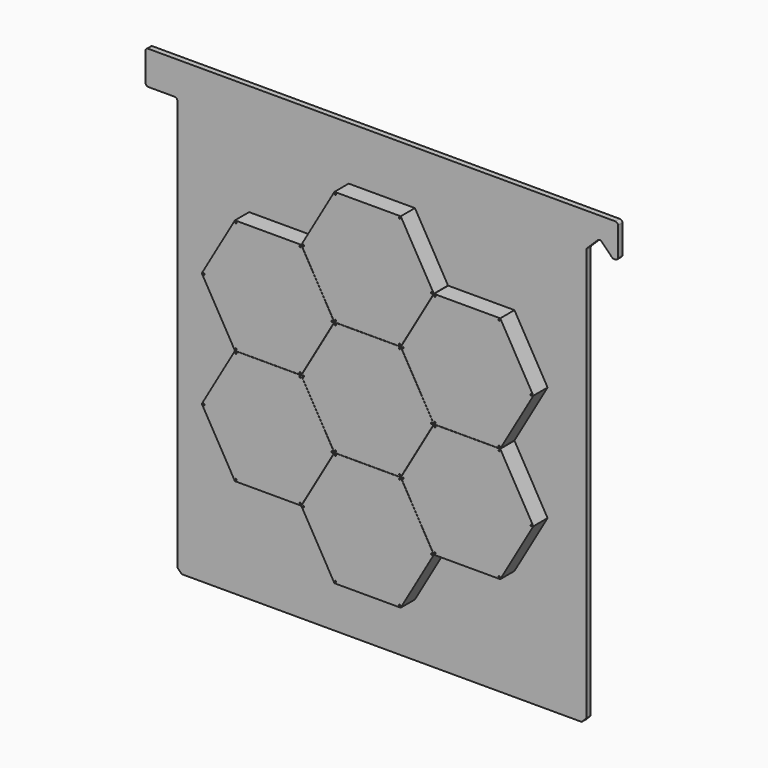
from build123d import *

# Parameters (mm, degrees)
F2_DEPTH = 6
F0_R     = 0.7500112
F0_R_2   = 0.7430174238
F3_DEPTH = 25.4


# Not quite as in the source:
# - ends of sketch curves that miss each other by under 0.0002 mm in the source are joined


with BuildPart() as f2:
    # F1 (on face) → F2 (new body)
    with BuildSketch(Plane.XZ):
        with BuildLine():
            Line((239.9250705835, 222.0849408719), (251.1754686974, 210.6445925623))
            ThreePointArc((251.1754686974, 210.6445925623), (252.1467535933, 209.9867437177), (253.2968294671, 209.755476289))
            Line((253.2968294671, 209.755476289), (254.8801768619, 209.755476289))
            ThreePointArc((254.8801768619, 209.755476289), (256.983999836, 210.6269082977), (257.8554318447, 212.7307312719))
            Line((257.8554318447, 212.7307312719), (257.8554318447, 243.475032761))
            ThreePointArc((257.8554318447, 243.475032761), (256.983999836, 245.5788557351), (254.8801768619, 246.4502877439))
            Line((254.8801768619, 246.4502877439), (-254.8801768619, 246.4502877439))
            ThreePointArc((-254.8801768619, 246.4502877439), (-256.983999836, 245.5788557351), (-257.8554318447, 243.475032761))
            Line((-257.8554318447, 243.475032761), (-257.8554318447, 212.7307312719))
            ThreePointArc((-257.8554318447, 212.7307312719), (-256.983999836, 210.6269082977), (-254.8801768619, 209.755476289))
            Line((-254.8801768619, 209.755476289), (-226.1193786946, 209.755476289))
            ThreePointArc((-226.1193786946, 209.755476289), (-224.0155557204, 208.8840442803), (-223.1441237117, 206.7802213062))
            Line((-223.1441237117, 206.7802213062), (-223.1441237117, -241.4915294391))
            Line((-223.1441237117, -241.4915294391), (-218.185365407, -246.4502877439))
            Line((-218.185365407, -246.4502877439), (218.185365407, -246.4502877439))
            Line((218.185365407, -246.4502877439), (223.1441237117, -241.4915294391))
            Line((223.1441237117, -241.4915294391), (223.1441237117, 208.5084705609))
            ThreePointArc((223.1441237117, 208.5084705609), (223.375391006, 209.658546114), (224.0332399627, 210.6298303616))
            Line((224.0332399627, 210.6298303616), (235.7175720959, 222.1201619404))
            ThreePointArc((235.7175720959, 222.1201619404), (237.8286155716, 222.9739529007), (239.9250705835, 222.0849408719))
        make_face()
        Polygon((72.2957914, 0), (36.1479084, -62.6100094), (-36.1479084, -62.6100094), (-72.2957914, 0), (-36.1479084, 62.6100094), (36.1479084, 62.6100094), align=None, mode=Mode.SUBTRACT)
    extrude(amount=F2_DEPTH)

    # F0 (on Front) → F3 (join)
    with BuildSketch(Plane.XZ):
        Polygon((36.1479084, -62.6100094), (72.2957914, 0), (36.1479084, 62.6100094), (-36.1479084, 62.6100094), (-72.2957914, 0), (-36.1479084, -62.6100094), align=None)
        with Locations((-34.993199, -60.609988)):
            Circle(F0_R, mode=Mode.SUBTRACT)
        with Locations((34.993199, -60.609988)):
            Circle(F0_R, mode=Mode.SUBTRACT)
        with Locations((-69.986398, 0)):
            Circle(F0_R, mode=Mode.SUBTRACT)
        with Locations((-34.993199, 60.609988)):
            Circle(F0_R, mode=Mode.SUBTRACT)
        with Locations((69.995796, 0)):
            Circle(F0_R_2, mode=Mode.SUBTRACT)
        with Locations((34.993199, 60.609988)):
            Circle(F0_R, mode=Mode.SUBTRACT)
        Polygon((72.47959348, -0.1061088931), (36.3364219227, -62.7188382077), (72.4890757311, -125.3261121412), (144.7848756936, -125.3206127679), (180.9280472508, -62.7078834532), (144.7753934424, -0.1006095197), align=None)
        with Locations((73.6436387774, -123.3260062512)):
            Circle(F0_R, mode=Mode.SUBTRACT)
        with Locations((143.6300274078, -123.3207069419)):
            Circle(F0_R, mode=Mode.SUBTRACT)
        with Locations((38.6458459563, -62.7186601398)):
            Circle(F0_R, mode=Mode.SUBTRACT)
        with Locations((73.6297421488, -2.0978761685)):
            Circle(F0_R_2, mode=Mode.SUBTRACT)
        with Locations((178.6186232172, -62.7080615211)):
            Circle(F0_R, mode=Mode.SUBTRACT)
        with Locations((143.6208303961, -2.1007154097)):
            Circle(F0_R, mode=Mode.SUBTRACT)
        Polygon((36.1478997424, -62.8259687739), (-36.1479168252, -62.8201722222), (-72.3008196697, -125.4272831471), (-36.1579567466, -188.0401906197), (36.1378598211, -188.0459871714), (72.2907626655, -125.4388762464), align=None)
        with Locations((-35.0030869921, -186.0402618087)):
            Circle(F0_R, mode=Mode.SUBTRACT)
        with Locations((-69.9914262771, -125.4274683102)):
            Circle(F0_R, mode=Mode.SUBTRACT)
        with Locations((-34.9933677872, -64.8202861983)):
            Circle(F0_R, mode=Mode.SUBTRACT)
        with Locations((34.983310783, -186.0458731952)):
            Circle(F0_R, mode=Mode.SUBTRACT)
        with Locations((69.9907672729, -125.4386918368)):
            Circle(F0_R_2, mode=Mode.SUBTRACT)
        with Locations((34.9930299879, -64.8258975849)):
            Circle(F0_R, mode=Mode.SUBTRACT)
        Polygon((-36.3200081195, -62.7093545109), (-72.4588066668, -0.0941010816), (-144.7546060688, -0.0835525132), (-180.91163233, -62.6883013644), (-144.7728337827, -125.3035547937), (-72.4770343807, -125.3141033621), align=None)
        with Locations((-143.6225460101, -123.3118678504)):
            Circle(F0_R_2, mode=Mode.SUBTRACT)
        with Locations((-73.6314577352, -123.3139168414)):
            Circle(F0_R, mode=Mode.SUBTRACT)
        with Locations((-178.6022083144, -62.6886407243)):
            Circle(F0_R, mode=Mode.SUBTRACT)
        with Locations((-143.6001827143, -2.0837390339)):
            Circle(F0_R, mode=Mode.SUBTRACT)
        with Locations((-38.6294321351, -62.709015151)):
            Circle(F0_R, mode=Mode.SUBTRACT)
        with Locations((-73.6137946247, -2.0939262472)):
            Circle(F0_R, mode=Mode.SUBTRACT)
        Polygon((-72.4855936704, 0.1095682125), (-36.3446929989, 62.7236083401), (-72.4996174478, 125.3295710344), (-144.7954171632, 125.3214496097), (-180.9363178347, 62.7074094821), (-144.7813933858, 0.1014467878), align=None)
        with Locations((-143.6269028809, 2.1015945506)):
            Circle(F0_R, mode=Mode.SUBTRACT)
        with Locations((-178.626893809, 62.707671309)):
            Circle(F0_R, mode=Mode.SUBTRACT)
        with Locations((-73.6405144887, 2.1094321527)):
            Circle(F0_R, mode=Mode.SUBTRACT)
        with Locations((-38.6541170246, 62.7233465131)):
            Circle(F0_R, mode=Mode.SUBTRACT)
        with Locations((-143.645196257, 123.3297240496)):
            Circle(F0_R_2, mode=Mode.SUBTRACT)
        with Locations((-73.6541079527, 123.3294232716)):
            Circle(F0_R, mode=Mode.SUBTRACT)
        Polygon((-36.1479091406, 62.8225415071), (36.1479076577, 62.8230453272), (72.2953543359, 125.4333066355), (36.1470350159, 188.0430641241), (-36.1487817824, 188.0425603041), (-72.2962284606, 125.4322989958), align=None)
        with Locations((-34.9932136785, 64.8225709541)):
            Circle(F0_R, mode=Mode.SUBTRACT)
        with Locations((-69.9868350606, 125.4323150896)):
            Circle(F0_R, mode=Mode.SUBTRACT)
        with Locations((-34.9940584445, 186.0425469512)):
            Circle(F0_R, mode=Mode.SUBTRACT)
        with Locations((34.9931843198, 64.8230586801)):
            Circle(F0_R, mode=Mode.SUBTRACT)
        with Locations((69.995358936, 125.4332906071)):
            Circle(F0_R_2, mode=Mode.SUBTRACT)
        with Locations((34.9923395538, 186.0430346772)):
            Circle(F0_R, mode=Mode.SUBTRACT)
        Polygon((36.3247836852, 62.71214389), (72.4809283845, 0.1069051082), (144.7767279344, 0.1163860718), (180.9164081792, 62.7311498147), (144.7602634799, 125.3363885966), (72.46446393, 125.3269076329), align=None)
        with Locations((73.6306643166, 2.098910662)):
            Circle(F0_R_2, mode=Mode.SUBTRACT)
        with Locations((38.6342077061, 62.7124443555)):
            Circle(F0_R, mode=Mode.SUBTRACT)
        with Locations((143.6217504731, 2.116252683)):
            Circle(F0_R, mode=Mode.SUBTRACT)
        with Locations((178.6069841582, 62.7308493493)):
            Circle(F0_R, mode=Mode.SUBTRACT)
        with Locations((73.6194413913, 123.3270410217)):
            Circle(F0_R, mode=Mode.SUBTRACT)
        with Locations((143.6058296174, 123.3362435186)):
            Circle(F0_R, mode=Mode.SUBTRACT)
    extrude(amount=F3_DEPTH)


solid = f2.part
